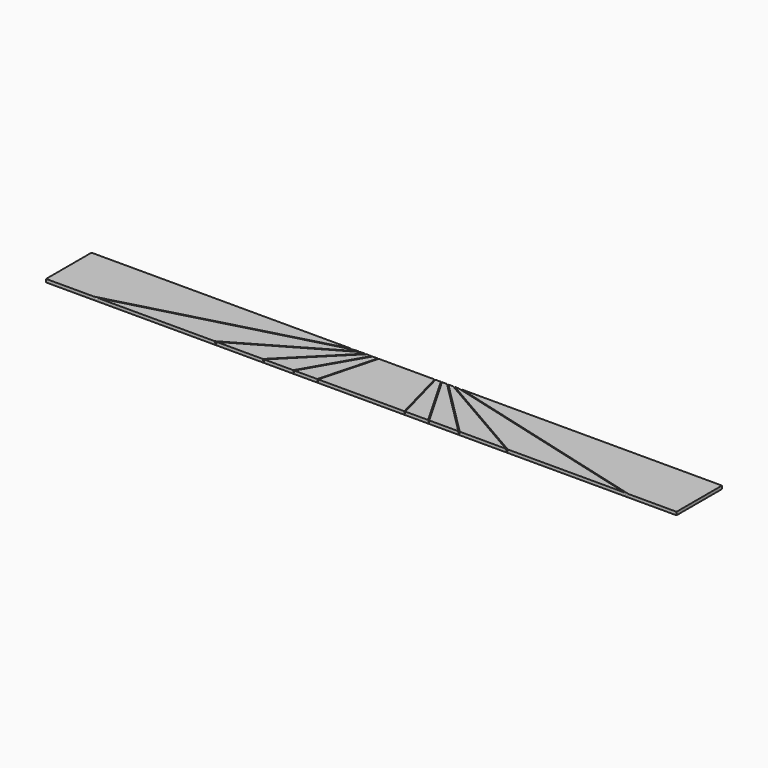
from build123d import *

# Parameters (mm, degrees)
F2_DEPTH    = 25.4
F3_DEPTH    = 25.4
F4_DEPTH    = 25.4
F5_DEPTH    = 25.4
F6_DEPTH    = 25.4
F7_DEPTH    = 25.4
F8_DEPTH    = 25.4
F9_DEPTH    = 25.4
F10_DEPTH   = 25.4
F11_DEPTH   = 25.4
F12_DEPTH   = 25.4
F13_SIZE2   = 4.022955
F13_SIZE    = 25.39999
F14_SIZE2   = 4.022955
F14_SIZE    = 25.39999
F14_2_SIZE2 = 4.022955
F14_2_SIZE  = 25.39999
F15_SIZE2   = 4.022955
F15_SIZE    = 25.39999
F15_2_SIZE2 = 4.022955
F15_2_SIZE  = 25.39999
F16_SIZE2   = 4.022955
F16_SIZE    = 25.39999
F16_2_SIZE2 = 4.022955
F16_2_SIZE  = 25.39999
F17_SIZE2   = 4.022955
F17_SIZE    = 25.39999
F17_2_SIZE2 = 4.022955
F17_2_SIZE  = 25.39999
F18_SIZE2   = 4.022955
F18_SIZE    = 25.39999
F18_2_SIZE2 = 4.022955
F18_2_SIZE  = 25.39999
F19_SIZE2   = 4.022955
F19_SIZE    = 25.39999
F19_2_SIZE2 = 4.022955
F19_2_SIZE  = 25.39999
F20_SIZE2   = 4.022955
F20_SIZE    = 25.39999
F20_2_SIZE2 = 4.022955
F20_2_SIZE  = 25.39999
F21_SIZE2   = 4.022955
F21_SIZE    = 25.39999
F21_2_SIZE2 = 4.022955
F21_2_SIZE  = 25.39999
F22_SIZE2   = 4.022955
F22_SIZE    = 25.39999
F22_2_SIZE2 = 4.022955
F22_2_SIZE  = 25.39999
F23_SIZE2   = 4.022955
F23_SIZE    = 25.39999


# Not quite as in the source:
# - a fillet or chamfer is up to 0.001 mm smaller than in the source, because OpenCascade refuses the exact size


with BuildPart() as f2:
    # F1 (on Top) → F2 (new body)
    with BuildSketch(Plane.XY):
        Polygon((-431.8, 228.6), (-2540, 228.6), (-2540, -228.6), (-2138.0936292205, -228.6), align=None)
    extrude(amount=F2_DEPTH)

    # F13 (size 25.4 and 4.0229647842 in the source; OpenCascade refuses exactly that, so slightly less here)
    f13_edges = [f2.edges().sort_by_distance(p)[0] for p in [
        (-1284.946815, 0, 25.4),
    ]]
    f13_side = f2.faces().sort_by_distance((-1284.946815, 0, 12.7))[0]
    chamfer(f13_edges, length=F13_SIZE, length2=F13_SIZE2, reference=f13_side)


with BuildPart() as f3:
    # F1 (on Top) → F3 (new body)
    with BuildSketch(Plane.XY):
        Polygon((-381, 228.6), (-431.8, 228.6), (-2138.0936292205, -228.6), (-1172.8936292205, -228.6), align=None)
    extrude(amount=F3_DEPTH)

    # F14 (size 25.4 and 4.0229647842 in the source; OpenCascade refuses exactly that, so slightly less here)
    f14_edges = [f3.edges().sort_by_distance(p)[0] for p in [
        (-1284.946815, 0, 25.4),
    ]]
    f14_side = f3.faces().sort_by_distance((-1284.946815, 0, 12.7))[0]
    chamfer(f14_edges, length=F14_SIZE, length2=F14_SIZE2, reference=f14_side)

    # F14#2 (size 25.4 and 4.0229647842 in the source; OpenCascade refuses exactly that, so slightly less here)
    f14_2_edges = [f3.edges().sort_by_distance(p)[0] for p in [
        (-776.946815, 0, 25.4),
    ]]
    f14_2_side = f3.faces().sort_by_distance((-776.946815, 0, 12.7))[0]
    chamfer(f14_2_edges, length=F14_2_SIZE, length2=F14_2_SIZE2, reference=f14_2_side)


with BuildPart() as f4:
    # F1 (on Top) → F4 (new body)
    with BuildSketch(Plane.XY):
        Polygon((-330.2, 228.6), (-381, 228.6), (-1172.8936292205, -228.6), (-787.4, -228.6), align=None)
    extrude(amount=F4_DEPTH)

    # F15 (size 25.4 and 4.0229647842 in the source; OpenCascade refuses exactly that, so slightly less here)
    f15_edges = [f4.edges().sort_by_distance(p)[0] for p in [
        (-776.946815, 0, 25.4),
    ]]
    f15_side = f4.faces().sort_by_distance((-776.946815, 0, 12.7))[0]
    chamfer(f15_edges, length=F15_SIZE, length2=F15_SIZE2, reference=f15_side)

    # F15#2 (size 25.4 and 4.0229647842 in the source; OpenCascade refuses exactly that, so slightly less here)
    f15_2_edges = [f4.edges().sort_by_distance(p)[0] for p in [
        (-558.8, 0, 25.4),
    ]]
    f15_2_side = f4.faces().sort_by_distance((-558.8, 0, 12.7))[0]
    chamfer(f15_2_edges, length=F15_2_SIZE, length2=F15_2_SIZE2, reference=f15_2_side)


with BuildPart() as f5:
    # F1 (on Top) → F5 (new body)
    with BuildSketch(Plane.XY):
        Polygon((-279.4, 228.6), (-330.2, 228.6), (-787.4, -228.6), (-543.3645430735, -228.6), align=None)
    extrude(amount=F5_DEPTH)

    # F16 (size 25.4 and 4.0229647842 in the source; OpenCascade refuses exactly that, so slightly less here)
    f16_edges = [f5.edges().sort_by_distance(p)[0] for p in [
        (-558.8, 0, 25.4),
    ]]
    f16_side = f5.faces().sort_by_distance((-558.8, 0, 12.7))[0]
    chamfer(f16_edges, length=F16_SIZE, length2=F16_SIZE2, reference=f16_side)

    # F16#2 (size 25.4 and 4.0229647842 in the source; OpenCascade refuses exactly that, so slightly less here)
    f16_2_edges = [f5.edges().sort_by_distance(p)[0] for p in [
        (-411.382272, 0, 25.4),
    ]]
    f16_2_side = f5.faces().sort_by_distance((-411.382272, 0, 12.7))[0]
    chamfer(f16_2_edges, length=F16_2_SIZE, length2=F16_2_SIZE2, reference=f16_2_side)


with BuildPart() as f6:
    # F1 (on Top) → F6 (new body)
    with BuildSketch(Plane.XY):
        Polygon((-228.6, 228.6), (-279.4, 228.6), (-543.3645430735, -228.6), (-351.1063707795, -228.6), align=None)
    extrude(amount=F6_DEPTH)

    # F17 (size 25.4 and 4.0229647842 in the source; OpenCascade refuses exactly that, so slightly less here)
    f17_edges = [f6.edges().sort_by_distance(p)[0] for p in [
        (-411.382272, 0, 25.4),
    ]]
    f17_side = f6.faces().sort_by_distance((-411.382272, 0, 12.7))[0]
    chamfer(f17_edges, length=F17_SIZE, length2=F17_SIZE2, reference=f17_side)

    # F17#2 (size 25.4 and 4.0229647842 in the source; OpenCascade refuses exactly that, so slightly less here)
    f17_2_edges = [f6.edges().sort_by_distance(p)[0] for p in [
        (-289.853185, 0, 25.4),
    ]]
    f17_2_side = f6.faces().sort_by_distance((-289.853185, 0, 12.7))[0]
    chamfer(f17_2_edges, length=F17_2_SIZE, length2=F17_2_SIZE2, reference=f17_2_side)


with BuildPart() as f7:
    # F1 (on Top) → F7 (new body)
    with BuildSketch(Plane.XY):
        Polygon((228.6, 228.6), (-228.6, 228.6), (-351.1063707795, -228.6), (351.1063707795, -228.6), align=None)
    extrude(amount=F7_DEPTH)

    # F18 (size 25.4 and 4.0229647842 in the source; OpenCascade refuses exactly that, so slightly less here)
    f18_edges = [f7.edges().sort_by_distance(p)[0] for p in [
        (-289.853185, 0, 25.4),
    ]]
    f18_side = f7.faces().sort_by_distance((-289.853185, 0, 12.7))[0]
    chamfer(f18_edges, length=F18_SIZE, length2=F18_SIZE2, reference=f18_side)

    # F18#2 (size 25.4 and 4.0229647842 in the source; OpenCascade refuses exactly that, so slightly less here)
    f18_2_edges = [f7.edges().sort_by_distance(p)[0] for p in [
        (289.853185, 0, 25.4),
    ]]
    f18_2_side = f7.faces().sort_by_distance((289.853185, 0, 12.7))[0]
    chamfer(f18_2_edges, length=F18_2_SIZE, length2=F18_2_SIZE2, reference=f18_2_side)


with BuildPart() as f8:
    # F1 (on Top) → F8 (new body)
    with BuildSketch(Plane.XY):
        Polygon((279.4, 228.6), (228.6, 228.6), (351.1063707795, -228.6), (543.3645430735, -228.6), align=None)
    extrude(amount=F8_DEPTH)

    # F19 (size 25.4 and 4.0229647842 in the source; OpenCascade refuses exactly that, so slightly less here)
    f19_edges = [f8.edges().sort_by_distance(p)[0] for p in [
        (289.853185, 0, 25.4),
    ]]
    f19_side = f8.faces().sort_by_distance((289.853185, 0, 12.7))[0]
    chamfer(f19_edges, length=F19_SIZE, length2=F19_SIZE2, reference=f19_side)

    # F19#2 (size 25.4 and 4.0229647842 in the source; OpenCascade refuses exactly that, so slightly less here)
    f19_2_edges = [f8.edges().sort_by_distance(p)[0] for p in [
        (411.382272, 0, 25.4),
    ]]
    f19_2_side = f8.faces().sort_by_distance((411.382272, 0, 12.7))[0]
    chamfer(f19_2_edges, length=F19_2_SIZE, length2=F19_2_SIZE2, reference=f19_2_side)


with BuildPart() as f9:
    # F1 (on Top) → F9 (new body)
    with BuildSketch(Plane.XY):
        Polygon((330.2, 228.6), (279.4, 228.6), (543.3645430735, -228.6), (787.4, -228.6), align=None)
    extrude(amount=F9_DEPTH)

    # F20 (size 25.4 and 4.0229647842 in the source; OpenCascade refuses exactly that, so slightly less here)
    f20_edges = [f9.edges().sort_by_distance(p)[0] for p in [
        (411.382272, 0, 25.4),
    ]]
    f20_side = f9.faces().sort_by_distance((411.382272, 0, 12.7))[0]
    chamfer(f20_edges, length=F20_SIZE, length2=F20_SIZE2, reference=f20_side)

    # F20#2 (size 25.4 and 4.0229647842 in the source; OpenCascade refuses exactly that, so slightly less here)
    f20_2_edges = [f9.edges().sort_by_distance(p)[0] for p in [
        (558.8, 0, 25.4),
    ]]
    f20_2_side = f9.faces().sort_by_distance((558.8, 0, 12.7))[0]
    chamfer(f20_2_edges, length=F20_2_SIZE, length2=F20_2_SIZE2, reference=f20_2_side)


with BuildPart() as f10:
    # F1 (on Top) → F10 (new body)
    with BuildSketch(Plane.XY):
        Polygon((381, 228.6), (330.2, 228.6), (787.4, -228.6), (1172.8936292205, -228.6), align=None)
    extrude(amount=F10_DEPTH)

    # F21 (size 25.4 and 4.0229647842 in the source; OpenCascade refuses exactly that, so slightly less here)
    f21_edges = [f10.edges().sort_by_distance(p)[0] for p in [
        (558.8, 0, 25.4),
    ]]
    f21_side = f10.faces().sort_by_distance((558.8, 0, 12.7))[0]
    chamfer(f21_edges, length=F21_SIZE, length2=F21_SIZE2, reference=f21_side)

    # F21#2 (size 25.4 and 4.0229647842 in the source; OpenCascade refuses exactly that, so slightly less here)
    f21_2_edges = [f10.edges().sort_by_distance(p)[0] for p in [
        (776.946815, 0, 25.4),
    ]]
    f21_2_side = f10.faces().sort_by_distance((776.946815, 0, 12.7))[0]
    chamfer(f21_2_edges, length=F21_2_SIZE, length2=F21_2_SIZE2, reference=f21_2_side)


with BuildPart() as f11:
    # F1 (on Top) → F11 (new body)
    with BuildSketch(Plane.XY):
        Polygon((431.8, 228.6), (381, 228.6), (1172.8936292205, -228.6), (2138.0936292205, -228.6), align=None)
    extrude(amount=F11_DEPTH)

    # F22 (size 25.4 and 4.0229647842 in the source; OpenCascade refuses exactly that, so slightly less here)
    f22_edges = [f11.edges().sort_by_distance(p)[0] for p in [
        (776.946815, 0, 25.4),
    ]]
    f22_side = f11.faces().sort_by_distance((776.946815, 0, 12.7))[0]
    chamfer(f22_edges, length=F22_SIZE, length2=F22_SIZE2, reference=f22_side)

    # F22#2 (size 25.4 and 4.0229647842 in the source; OpenCascade refuses exactly that, so slightly less here)
    f22_2_edges = [f11.edges().sort_by_distance(p)[0] for p in [
        (1284.946815, 0, 25.4),
    ]]
    f22_2_side = f11.faces().sort_by_distance((1284.946815, 0, 12.7))[0]
    chamfer(f22_2_edges, length=F22_2_SIZE, length2=F22_2_SIZE2, reference=f22_2_side)


with BuildPart() as f12:
    # F1 (on Top) → F12 (new body)
    with BuildSketch(Plane.XY):
        Polygon((2540, 228.6), (431.8, 228.6), (2138.0936292205, -228.6), (2540, -228.6), align=None)
    extrude(amount=F12_DEPTH)

    # F23 (size 25.4 and 4.0229647842 in the source; OpenCascade refuses exactly that, so slightly less here)
    f23_edges = [f12.edges().sort_by_distance(p)[0] for p in [
        (1284.946815, 0, 25.4),
    ]]
    f23_side = f12.faces().sort_by_distance((1284.946815, 0, 12.7))[0]
    chamfer(f23_edges, length=F23_SIZE, length2=F23_SIZE2, reference=f23_side)


solid = Compound([f2.part, f3.part, f4.part, f5.part, f6.part, f7.part, f8.part, f9.part, f10.part, f11.part, f12.part])
